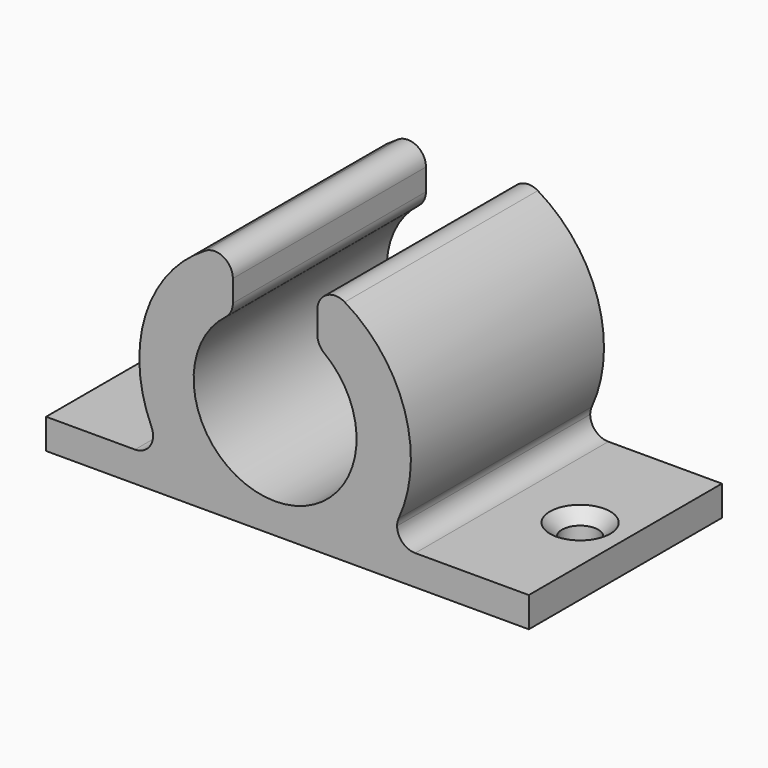
from build123d import *

# Parameters (mm, degrees)
F0_W        = 80
F0_H        = 40
F0_R        = 3
F0_W_2      = 50
F0_H_2      = 30
F1_DEPTH    = 5
F2_SIZE     = 2
F6_DEPTH    = 40
F7_T1_DEPTH = 40
F7_T3_DEPTH = 64.9354908843
F7_T5_DEPTH = 47.905041839


# Not quite as in the source:
# - a fillet or chamfer that OpenCascade refuses, or shapes differently, is made with other operations: its cross-section is extruded or revolved along the edge and cut away or added


with BuildPart() as f1:
    # F0 (on Top) → F1 (new body)
    with BuildSketch(Plane.XY):
        with Locations((40, -20)):
            Rectangle(F0_W, F0_H)
        with Locations((7.5, -20)):
            Circle(F0_R, mode=Mode.SUBTRACT)
        with Locations((40, -20)):
            Rectangle(F0_W_2, F0_H_2, mode=Mode.SUBTRACT)
        with Locations((72.5, -20)):
            Circle(F0_R, mode=Mode.SUBTRACT)
        with Locations((40, -20)):
            Rectangle(F0_W_2, F0_H_2)
    extrude(amount=F1_DEPTH)

    # F2
    f2_edges = [f1.edges().sort_by_distance(p)[0] for p in [
        (4.5, -20, 5),
        (69.5, -20, 5),
    ]]
    chamfer(f2_edges, length=F2_SIZE)

    # F5 (on plane+point) → F6 (join)
    with BuildSketch(Plane(origin=(0, 0, 0), x_dir=(-1, 0, 0), z_dir=(0, 1, 0))):
        with BuildLine():
            ThreePointArc((-30.954095751, 30.0433963806), (-37.954095751, 5), (-44.954095751, 30.0433963806))
            Line((-44.954095751, 30.0433963806), (-44.954095751, 39.8834047803))
            ThreePointArc((-44.954095751, 39.8834047803), (-58.6775836128, 27.2628220822), (-58.1714250849, 8.625305341))
            Line((-58.1714250849, 8.625305341), (-58.1714250849, 0))
            Line((-58.1714250849, 0), (-17.7367664172, 0))
            Line((-17.7367664172, 0), (-17.7367664172, 8.625305341))
            ThreePointArc((-17.7367664172, 8.625305341), (-17.2306078893, 27.2628220822), (-30.954095751, 39.8834047803))
            Line((-30.954095751, 39.8834047803), (-30.954095751, 30.0433963806))
        make_face()
    extrude(amount=-F6_DEPTH)

    # F7: fillet of radius 3 on 8 edges, made by hand

    # F7_s2 → F7_t1 (join)
    with BuildSketch(Plane.XZ):
        with BuildLine():
            ThreePointArc((58.1714250849, 7.9545925349), (58.2393309928, 8.5892768936), (58.439974575, 9.1952287073))
            ThreePointArc((58.439974575, 9.1952287073), (58.3076947386, 8.9093270176), (58.1714250849, 8.625305341))
            Line((58.1714250849, 8.625305341), (58.1714250849, 7.9545925349))
        make_face()
        with BuildLine():
            ThreePointArc((61.1714250849, 5), (59.0501047413, 5.8786796564), (58.1714250849, 8))
            Line((58.1714250849, 8), (58.1714250849, 5))
            Line((58.1714250849, 5), (61.1714250849, 5))
        make_face()
        with BuildLine():
            ThreePointArc((17.4682169271, 9.1952287073), (17.6688605093, 8.5892768936), (17.7367664172, 7.9545925349))
            Line((17.7367664172, 7.9545925349), (17.7367664172, 8.625305341))
            ThreePointArc((17.7367664172, 8.625305341), (17.6004967635, 8.9093270176), (17.4682169271, 9.1952287073))
        make_face()
        with BuildLine():
            ThreePointArc((17.7367664172, 8), (16.8580867608, 5.8786796564), (14.7367664172, 5))
            Line((14.7367664172, 5), (17.7367664172, 5))
            Line((17.7367664172, 5), (17.7367664172, 8))
        make_face()
    extrude(amount=F7_T1_DEPTH)

    # F7_s4 → F7_t3 (cut)
    with BuildSketch(Plane.XZ.offset(-12.4677454421)):
        with BuildLine():
            ThreePointArc((44.954095751, 35.2406690428), (46.4734514007, 37.8498245207), (49.4925572895, 37.8161565878))
            ThreePointArc((49.4925572895, 37.8161565878), (47.2807788606, 38.9759122428), (44.954095751, 39.8834047803))
            Line((44.954095751, 39.8834047803), (44.954095751, 35.2406690428))
        make_face()
        with BuildLine():
            ThreePointArc((26.4156342126, 37.8161565878), (29.4347401014, 37.8498245207), (30.954095751, 35.2406690428))
            Line((30.954095751, 35.2406690428), (30.954095751, 39.8834047803))
            ThreePointArc((30.954095751, 39.8834047803), (28.6274126415, 38.9759122428), (26.4156342126, 37.8161565878))
        make_face()
    extrude(amount=F7_T3_DEPTH, mode=Mode.SUBTRACT)

    # F7_s6 → F7_t5 (cut)
    with BuildSketch(Plane.XZ.offset(-3.9525209195)):
        with BuildLine():
            ThreePointArc((46.1359139329, 29.2381493396), (45.2657370088, 30.2929667015), (44.954095751, 31.6244047484))
            Line((44.954095751, 31.6244047484), (44.954095751, 30.0433963806))
            ThreePointArc((44.954095751, 30.0433963806), (45.5556749637, 29.6564328293), (46.1359139329, 29.2381493396))
        make_face()
        with BuildLine():
            ThreePointArc((30.954095751, 31.6244047484), (30.6424544933, 30.2929667015), (29.7722775692, 29.2381493396))
            ThreePointArc((29.7722775692, 29.2381493396), (30.3525165384, 29.6564328293), (30.954095751, 30.0433963806))
            Line((30.954095751, 30.0433963806), (30.954095751, 31.6244047484))
        make_face()
    extrude(amount=F7_T5_DEPTH, mode=Mode.SUBTRACT)


solid = f1.part
